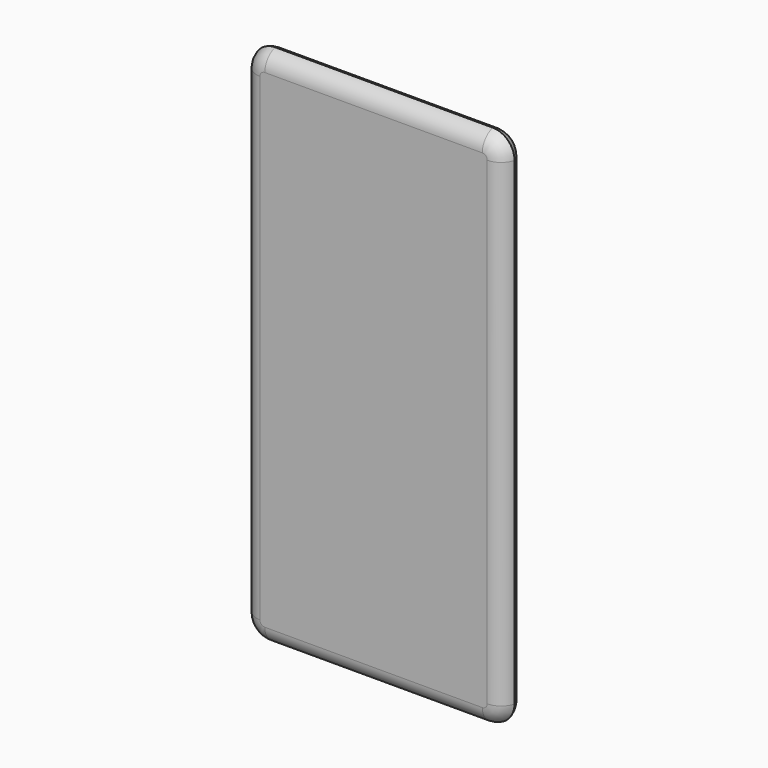
from build123d import *

# Parameters (mm, degrees)
F1_DEPTH     = 3.81
F2_T1_DEPTH  = 139.7
F2_T3_DEPTH  = 63.5
F2_T6_ANGLE  = 90
F2_T8_ANGLE  = 90
F2_T10_ANGLE = 90
F2_T12_ANGLE = 90
F3_DEPTH     = 3.81
F4_T1_DEPTH  = 139.7
F4_T3_DEPTH  = 63.5
F4_T6_ANGLE  = 90
F4_T8_ANGLE  = 90
F4_T10_ANGLE = 90
F4_T12_ANGLE = 90


# Not quite as in the source:
# - a fillet or chamfer that OpenCascade refuses, or shapes differently, is made with other operations: its cross-section is extruded or revolved along the edge and cut away or added
# - the program builds the solid bodies; features that only make, move or delete a surface that nothing else refers to are left out


with BuildPart() as f1:
    # F0 (on Front) → F1 (new body)
    with BuildSketch(Plane.XZ):
        with BuildLine():
            Line((-31.75, -76.2), (31.75, -76.2))
            ThreePointArc((31.75, -76.2), (36.2401280605, -74.3401280605), (38.1, -69.85))
            Line((38.1, -69.85), (38.1, 69.85))
            ThreePointArc((38.1, 69.85), (36.2401280605, 74.3401280605), (31.75, 76.2))
            Line((31.75, 76.2), (-31.75, 76.2))
            ThreePointArc((-31.75, 76.2), (-36.2401280605, 74.3401280605), (-38.1, 69.85))
            Line((-38.1, 69.85), (-38.1, -69.85))
            ThreePointArc((-38.1, -69.85), (-36.2401280605, -74.3401280605), (-31.75, -76.2))
        make_face()
    extrude(amount=F1_DEPTH)

    # F2: fillet of radius 5.08 on 1 edges, made by hand

    # F2_s2 → F2_t1 (cut)
    with BuildSketch(Plane.XY.offset(-69.85)):
        with BuildLine():
            ThreePointArc((38.1, 0), (36.2921631237, -2.7460926284), (33.1813111503, -3.81))
            Line((33.1813111503, -3.81), (38.1, -3.81))
            Line((38.1, -3.81), (38.1, 0))
        make_face()
        with BuildLine():
            ThreePointArc((-38.1, 0), (-36.2921631237, -2.7460926284), (-33.1813111503, -3.81))
            Line((-33.1813111503, -3.81), (-38.1, -3.81))
            Line((-38.1, -3.81), (-38.1, 0))
        make_face()
    extrude(amount=F2_T1_DEPTH, mode=Mode.SUBTRACT)

    # F2_s4 → F2_t3 (cut)
    with BuildSketch(Plane.YZ.offset(-31.75)):
        with BuildLine():
            ThreePointArc((0, 76.2), (-2.7460926284, 74.3921631237), (-3.81, 71.2813111503))
            Line((-3.81, 71.2813111503), (-3.81, 76.2))
            Line((-3.81, 76.2), (0, 76.2))
        make_face()
        with BuildLine():
            ThreePointArc((0, -76.2), (-2.7460926284, -74.3921631237), (-3.81, -71.2813111503))
            Line((-3.81, -71.2813111503), (-3.81, -76.2))
            Line((-3.81, -76.2), (0, -76.2))
        make_face()
    extrude(amount=F2_T3_DEPTH, mode=Mode.SUBTRACT)

    # F2_s5 → F2_t6 (revolve, cut)
    with BuildSketch(Plane.YZ.offset(31.75)):
        with BuildLine():
            ThreePointArc((0, -76.2), (-2.7460926284, -74.3921631237), (-3.81, -71.2813111503))
            Line((-3.81, -71.2813111503), (-3.81, -76.2))
            Line((-3.81, -76.2), (0, -76.2))
        make_face()
    revolve(axis=Axis((31.75, -3.81, -69.85), (0, -1, 0)), revolution_arc=F2_T6_ANGLE, mode=Mode.SUBTRACT)

    # F2_s7 → F2_t8 (revolve, cut)
    with BuildSketch(Plane.XY.offset(69.85)):
        with BuildLine():
            ThreePointArc((38.1, 0), (36.2921631237, -2.7460926284), (33.1813111503, -3.81))
            Line((33.1813111503, -3.81), (38.1, -3.81))
            Line((38.1, -3.81), (38.1, 0))
        make_face()
    revolve(axis=Axis((31.75, -3.81, 69.85), (0, -1, 0)), revolution_arc=F2_T8_ANGLE, mode=Mode.SUBTRACT)

    # F2_s9 → F2_t10 (revolve, cut)
    with BuildSketch(Plane.YZ.offset(-31.75)):
        with BuildLine():
            ThreePointArc((0, 76.2), (-2.7460926284, 74.3921631237), (-3.81, 71.2813111503))
            Line((-3.81, 71.2813111503), (-3.81, 76.2))
            Line((-3.81, 76.2), (0, 76.2))
        make_face()
    revolve(axis=Axis((-31.75, -3.81, 69.85), (0, -1, 0)), revolution_arc=F2_T10_ANGLE, mode=Mode.SUBTRACT)

    # F2_s11 → F2_t12 (revolve, cut)
    with BuildSketch(Plane.XY.offset(-69.85)):
        with BuildLine():
            ThreePointArc((-38.1, 0), (-36.2921631237, -2.7460926284), (-33.1813111503, -3.81))
            Line((-33.1813111503, -3.81), (-38.1, -3.81))
            Line((-38.1, -3.81), (-38.1, 0))
        make_face()
    revolve(axis=Axis((-31.75, -3.81, -69.85), (0, -1, 0)), revolution_arc=F2_T12_ANGLE, mode=Mode.SUBTRACT)

    # F3 (add): a face of the model
    f3_faces = [f1.faces().sort_by_distance(p)[0] for p in [
        (0, 0, 0),
    ]]
    extrude(f3_faces, amount=F3_DEPTH)

    # F4: fillet of radius 5.08 on 1 edges, made by hand

    # F4_s2 → F4_t1 (cut)
    with BuildSketch(Plane.XY.offset(-69.85)):
        with BuildLine():
            ThreePointArc((33.1813111503, 3.81), (36.2921631237, 2.7460926284), (38.1, 0))
            Line((38.1, 0), (38.1, 3.81))
            Line((38.1, 3.81), (33.1813111503, 3.81))
        make_face()
        with BuildLine():
            ThreePointArc((-38.1, 0), (-36.2921631237, 2.7460926284), (-33.1813111503, 3.81))
            Line((-33.1813111503, 3.81), (-38.1, 3.81))
            Line((-38.1, 3.81), (-38.1, 0))
        make_face()
    extrude(amount=F4_T1_DEPTH, mode=Mode.SUBTRACT)

    # F4_s4 → F4_t3 (cut)
    with BuildSketch(Plane.YZ.offset(-31.75)):
        with BuildLine():
            ThreePointArc((3.81, 71.2813111503), (2.7460926284, 74.3921631237), (0, 76.2))
            Line((0, 76.2), (3.81, 76.2))
            Line((3.81, 76.2), (3.81, 71.2813111503))
        make_face()
        with BuildLine():
            ThreePointArc((3.81, -71.2813111503), (2.7460926284, -74.3921631237), (0, -76.2))
            Line((0, -76.2), (3.81, -76.2))
            Line((3.81, -76.2), (3.81, -71.2813111503))
        make_face()
    extrude(amount=F4_T3_DEPTH, mode=Mode.SUBTRACT)

    # F4_s5 → F4_t6 (revolve, cut)
    with BuildSketch(Plane.YZ.offset(31.75)):
        with BuildLine():
            ThreePointArc((3.81, -71.2813111503), (2.7460926284, -74.3921631237), (0, -76.2))
            Line((0, -76.2), (3.81, -76.2))
            Line((3.81, -76.2), (3.81, -71.2813111503))
        make_face()
    revolve(axis=Axis((31.75, 3.81, -69.85), (0, -1, 0)), revolution_arc=F4_T6_ANGLE, mode=Mode.SUBTRACT)

    # F4_s7 → F4_t8 (revolve, cut)
    with BuildSketch(Plane.XY.offset(69.85)):
        with BuildLine():
            ThreePointArc((33.1813111503, 3.81), (36.2921631237, 2.7460926284), (38.1, 0))
            Line((38.1, 0), (38.1, 3.81))
            Line((38.1, 3.81), (33.1813111503, 3.81))
        make_face()
    revolve(axis=Axis((31.75, 3.81, 69.85), (0, -1, 0)), revolution_arc=F4_T8_ANGLE, mode=Mode.SUBTRACT)

    # F4_s9 → F4_t10 (revolve, cut)
    with BuildSketch(Plane.YZ.offset(-31.75)):
        with BuildLine():
            ThreePointArc((0, 76.2), (2.7460926284, 74.3921631237), (3.81, 71.2813111503))
            Line((3.81, 71.2813111503), (3.81, 76.2))
            Line((3.81, 76.2), (0, 76.2))
        make_face()
    revolve(axis=Axis((-31.75, 3.81, 69.85), (0, -1, 0)), revolution_arc=F4_T10_ANGLE, mode=Mode.SUBTRACT)

    # F4_s11 → F4_t12 (revolve, cut)
    with BuildSketch(Plane.XY.offset(-69.85)):
        with BuildLine():
            ThreePointArc((-38.1, 0), (-36.2921631237, 2.7460926284), (-33.1813111503, 3.81))
            Line((-33.1813111503, 3.81), (-38.1, 3.81))
            Line((-38.1, 3.81), (-38.1, 0))
        make_face()
    revolve(axis=Axis((-31.75, 3.81, -69.85), (0, -1, 0)), revolution_arc=F4_T12_ANGLE, mode=Mode.SUBTRACT)


solid = f1.part
